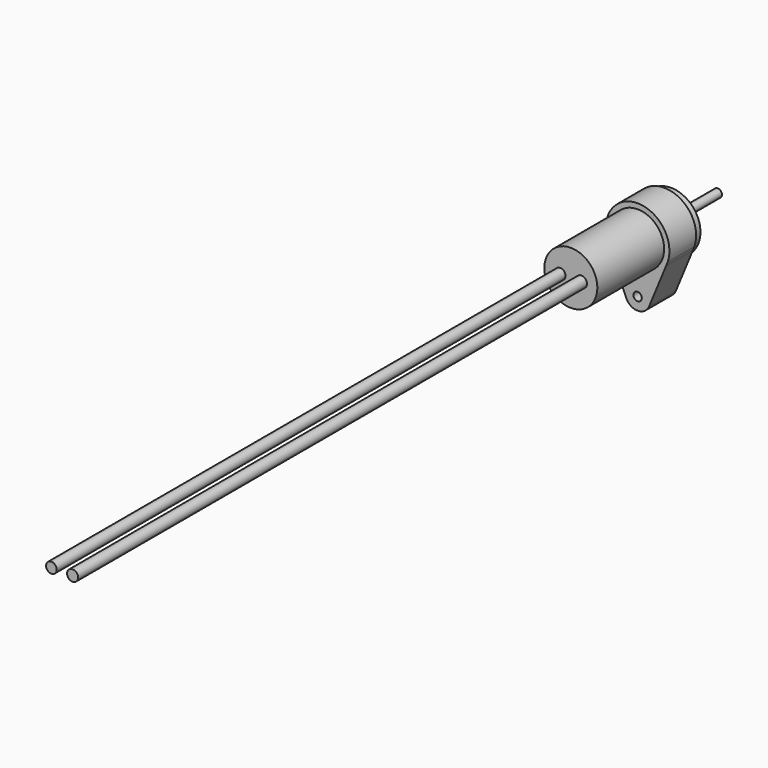
from build123d import *

# Parameters (mm, degrees)
F0_R     = 3.175
F1_DEPTH = 15
F2_R     = 0.5
F3_DEPTH = 7
F4_R     = 0.5
F4_R_2   = 3.175
F5_DEPTH = 5
F6_R     = 9.3189524644
F6_R_2   = 3.5292713956
F7_DEPTH = 1
F8_R     = 0.635
F8_R_2   = 0.6612583991
F9_DEPTH = 76.2


with BuildPart() as f1:
    # F0 (on Front) → F1 (new body)
    with BuildSketch(Plane.XZ):
        Circle(F0_R)
    extrude(amount=F1_DEPTH)

    # F2 (on face) → F3 (join)
    with BuildSketch(Plane(origin=(0, 0, 0), x_dir=(-1, 0, 0), z_dir=(0, 1, 0))):
        Circle(F2_R)
    extrude(amount=F3_DEPTH)

    # F4 (on face) → F5 (join)
    with BuildSketch(Plane(origin=(0, 0, 0), x_dir=(-1, 0, 0), z_dir=(0, 1, 0))):
        with BuildLine():
            Line((1.3866466063, -6.6022387167), (3.4052943148, -1.7088214153))
            Line((3.4052943148, -1.7088214153), (3.6196746552, -1.1891406101))
            ThreePointArc((3.6196746552, -1.1891406101), (0, 3.81), (-3.6196746552, -1.1891406101))
            Line((-3.6196746552, -1.1891406101), (-3.4052943148, -1.7088214153))
            Line((-3.4052943148, -1.7088214153), (-1.3866466063, -6.6022387167))
            ThreePointArc((-1.3866466063, -6.6022387167), (0, -7.5302149504), (1.3866466063, -6.6022387167))
        make_face()
        with Locations((0, -6.0302149504)):
            Circle(F4_R, mode=Mode.SUBTRACT)
        Circle(F4_R_2, mode=Mode.SUBTRACT)
        Circle(F4_R_2)
        Circle(F4_R, mode=Mode.SUBTRACT)
    extrude(amount=-F5_DEPTH)

    # F6 (on face) → F7 (cut)
    with BuildSketch(Plane(origin=(0, 0, 0), x_dir=(-1, 0, 0), z_dir=(0, 1, 0))):
        Circle(F6_R)
        with Locations((0, -0.1206563757)):
            Circle(F6_R_2, mode=Mode.SUBTRACT)
    extrude(amount=-F7_DEPTH, mode=Mode.SUBTRACT)

    # F8 (on face) → F9 (join)
    with BuildSketch(Plane.XZ.offset(15)):
        with Locations((-1.27, 0)):
            Circle(F8_R)
        with Locations((1.27, 0)):
            Circle(F8_R_2)
    extrude(amount=F9_DEPTH)


solid = f1.part
